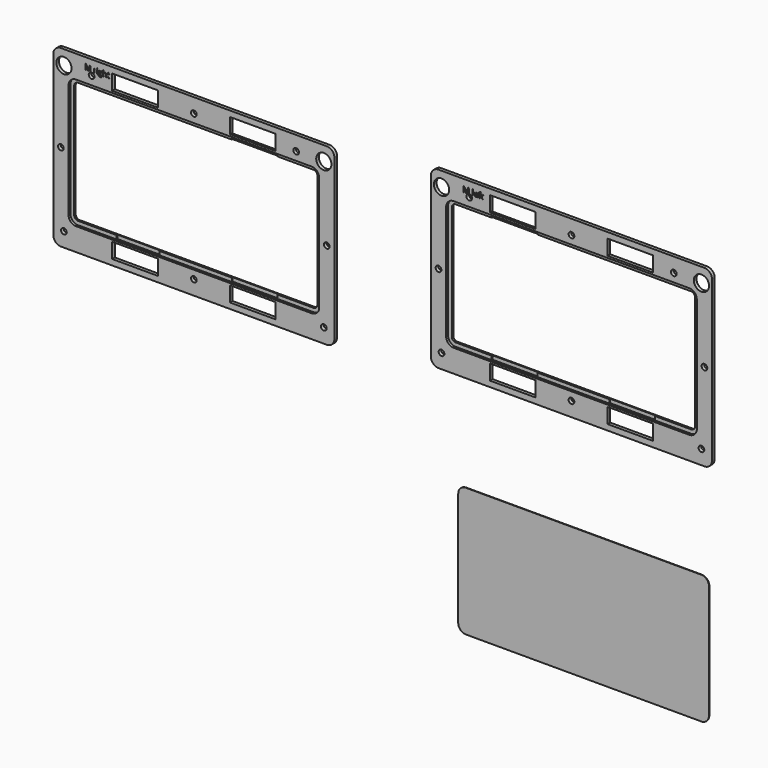
from build123d import *

# Parameters (mm, degrees)
F0_R          = 2.38125
F0_W          = 38.1
F0_H          = 12.7
F0_R_2        = 6.35
F0_R_3        = 2.3876
F1_DEPTH      = 0.79375
F2_R          = 2.38125
F2_W          = 38.1
F2_H          = 12.7
F2_R_2        = 6.35
F2_R_3        = 2.3876
F3_DEPTH      = 1.984375
F5_DEPTH      = 0.396875
F7_DEPTH      = 0.79375
F8_W          = 38.121374324
F8_H          = 5.2950307727
F9_DEPTH      = 0.79375
F10_TEXT_SIZE = 6.5434620612
F11_DEPTH     = 0.396875
F12_R         = 2.38125
F12_W         = 38.1
F12_H         = 12.7
F12_R_2       = 6.35
F12_R_3       = 2.3876
F13_DEPTH     = 0.79375
F14_R         = 2.38125
F14_W         = 38.1
F14_H         = 12.7
F14_R_2       = 6.35
F14_R_3       = 2.3876
F15_DEPTH     = 1.984375
F16_TEXT_SIZE = 6.2933967759
F17_DEPTH     = 0.396875
F19_DEPTH     = 0.79375
F20_W         = 38.1
F20_H         = 7.678820458
F20_H_2       = 9.2029287548
F20_W_2       = 35.9697821996
F20_H_3       = 10.6201223166
F21_DEPTH     = 0.79375


# Not quite as in the source:
# - Text() gives the source's letters only with a copy of the font that has no kerning and outlines rounded to 1/6400 em; it was checked with that copy


with BuildPart() as f1:
    # F0 (on Front) → F1 (new body)
    with BuildSketch(Plane.XZ):
        with BuildLine():
            Line((124.1159564874, 73.3042017429), (-98.1340435126, 73.3042017429))
            ThreePointArc((-98.1340435126, 73.3042017429), (-102.6241715732, 71.4443298034), (-104.4840435126, 66.9542017429))
            Line((-104.4840435126, 66.9542017429), (-104.4840435126, -66.3957982571))
            ThreePointArc((-104.4840435126, -66.3957982571), (-102.6241715732, -70.8859263176), (-98.1340435126, -72.7457982571))
            Line((-98.1340435126, -72.7457982571), (124.1159564874, -72.7457982571))
            ThreePointArc((124.1159564874, -72.7457982571), (128.6060845479, -70.8859263176), (130.4659564874, -66.3957982571))
            Line((130.4659564874, -66.3957982571), (130.4659564874, 66.9542017429))
            ThreePointArc((130.4659564874, 66.9542017429), (128.6060845479, 71.4443298034), (124.1159564874, 73.3042017429))
        make_face()
        with Locations((-95.6166075429, -60.7033622874)):
            Circle(F0_R, mode=Mode.SUBTRACT)
        with Locations((-36.2215435126, -61.6332982571)):
            Rectangle(F0_W, F0_H, mode=Mode.SUBTRACT)
        with Locations((12.994937633, -60.7033622874)):
            Circle(F0_R, mode=Mode.SUBTRACT)
        with Locations((62.2034564874, -61.6332982571)):
            Rectangle(F0_W, F0_H, mode=Mode.SUBTRACT)
        with Locations((121.5985205176, -60.7033622874)):
            Circle(F0_R, mode=Mode.SUBTRACT)
        with Locations((-98.1340435126, 0.2792017429)):
            Circle(F0_R, mode=Mode.SUBTRACT)
        with BuildLine():
            ThreePointArc((-91.7840435126, 47.9042017429), (-89.9241715732, 52.3943298034), (-85.4340435126, 54.2542017429))
            Line((-85.4340435126, 54.2542017429), (111.4159564874, 54.2542017429))
            ThreePointArc((111.4159564874, 54.2542017429), (115.9060845479, 52.3943298034), (117.7659564874, 47.9042017429))
            Line((117.7659564874, 47.9042017429), (117.7659564874, -47.3457982571))
            ThreePointArc((117.7659564874, -47.3457982571), (115.9060845479, -51.8359263176), (111.4159564874, -53.6957982571))
            Line((111.4159564874, -53.6957982571), (-85.4340435126, -53.6957982571))
            ThreePointArc((-85.4340435126, -53.6957982571), (-89.9241715732, -51.8359263176), (-91.7840435126, -47.3457982571))
            Line((-91.7840435126, -47.3457982571), (-91.7840435126, 47.9042017429))
        make_face(mode=Mode.SUBTRACT)
        with Locations((-95.6166075429, 61.2617657732)):
            Circle(F0_R_2, mode=Mode.SUBTRACT)
        with Locations((-72.4865459126, 61.2617657732)):
            Circle(F0_R_3, mode=Mode.SUBTRACT)
        with Locations((-36.2215435126, 62.1917017429)):
            Rectangle(F0_W, F0_H, mode=Mode.SUBTRACT)
        with Locations((124.1159564874, 0.2792017429)):
            Circle(F0_R, mode=Mode.SUBTRACT)
        with Locations((12.994937633, 61.2617657732)):
            Circle(F0_R, mode=Mode.SUBTRACT)
        with Locations((62.2034564874, 62.1917017429)):
            Rectangle(F0_W, F0_H, mode=Mode.SUBTRACT)
        with Locations((98.4684588874, 61.2617657732)):
            Circle(F0_R_3, mode=Mode.SUBTRACT)
        with Locations((121.5985205176, 61.2617657732)):
            Circle(F0_R_2, mode=Mode.SUBTRACT)
        with BuildLine():
            Line((111.4159564874, 54.2542017429), (-85.4340435126, 54.2542017429))
            ThreePointArc((-85.4340435126, 54.2542017429), (-89.9241715732, 52.3943298034), (-91.7840435126, 47.9042017429))
            Line((-91.7840435126, 47.9042017429), (-91.7840435126, -47.3457982571))
            ThreePointArc((-91.7840435126, -47.3457982571), (-89.9241715732, -51.8359263176), (-85.4340435126, -53.6957982571))
            Line((-85.4340435126, -53.6957982571), (111.4159564874, -53.6957982571))
            ThreePointArc((111.4159564874, -53.6957982571), (115.9060845479, -51.8359263176), (117.7659564874, -47.3457982571))
            Line((117.7659564874, -47.3457982571), (117.7659564874, 47.9042017429))
            ThreePointArc((117.7659564874, 47.9042017429), (115.9060845479, 52.3943298034), (111.4159564874, 54.2542017429))
        make_face()
        with BuildLine():
            ThreePointArc((-88.6090435126, 47.9042017429), (-87.6791075429, 50.1492657732), (-85.4340435126, 51.0792017429))
            Line((-85.4340435126, 51.0792017429), (111.4159564874, 51.0792017429))
            ThreePointArc((111.4159564874, 51.0792017429), (113.6610205176, 50.1492657732), (114.5909564874, 47.9042017429))
            Line((114.5909564874, 47.9042017429), (114.5909564874, -47.3457982571))
            ThreePointArc((114.5909564874, -47.3457982571), (113.6610205176, -49.5908622874), (111.4159564874, -50.5207982571))
            Line((111.4159564874, -50.5207982571), (-85.4340435126, -50.5207982571))
            ThreePointArc((-85.4340435126, -50.5207982571), (-87.6791075429, -49.5908622874), (-88.6090435126, -47.3457982571))
            Line((-88.6090435126, -47.3457982571), (-88.6090435126, 47.9042017429))
        make_face(mode=Mode.SUBTRACT)
    extrude(amount=F1_DEPTH)

    # F2 (on face) → F3 (join)
    with BuildSketch(Plane.XZ.offset(0.79375)):
        with BuildLine():
            ThreePointArc((124.1159564874, -72.7457982571), (128.6060845479, -70.8859263176), (130.4659564874, -66.3957982571))
            Line((130.4659564874, -66.3957982571), (130.4659564874, 66.9542017429))
            ThreePointArc((130.4659564874, 66.9542017429), (128.6060845479, 71.4443298034), (124.1159564874, 73.3042017429))
            Line((124.1159564874, 73.3042017429), (-98.1340435126, 73.3042017429))
            ThreePointArc((-98.1340435126, 73.3042017429), (-102.6241715732, 71.4443298034), (-104.4840435126, 66.9542017429))
            Line((-104.4840435126, 66.9542017429), (-104.4840435126, -66.3957982571))
            ThreePointArc((-104.4840435126, -66.3957982571), (-102.6241715732, -70.8859263176), (-98.1340435126, -72.7457982571))
            Line((-98.1340435126, -72.7457982571), (124.1159564874, -72.7457982571))
        make_face()
        with Locations((-95.6166075429, -60.7033622874)):
            Circle(F2_R, mode=Mode.SUBTRACT)
        with Locations((-36.2215435126, -61.6332982571)):
            Rectangle(F2_W, F2_H, mode=Mode.SUBTRACT)
        with Locations((12.994937633, -60.7033622874)):
            Circle(F2_R, mode=Mode.SUBTRACT)
        with Locations((62.2034564874, -61.6332982571)):
            Rectangle(F2_W, F2_H, mode=Mode.SUBTRACT)
        with Locations((121.5985205176, -60.7033622874)):
            Circle(F2_R, mode=Mode.SUBTRACT)
        with Locations((-98.1340435126, 0.2792017429)):
            Circle(F2_R, mode=Mode.SUBTRACT)
        with BuildLine():
            ThreePointArc((-91.7840435126, 47.9042017429), (-89.9241715732, 52.3943298034), (-85.4340435126, 54.2542017429))
            Line((-85.4340435126, 54.2542017429), (111.4159564874, 54.2542017429))
            ThreePointArc((111.4159564874, 54.2542017429), (115.9060845479, 52.3943298034), (117.7659564874, 47.9042017429))
            Line((117.7659564874, 47.9042017429), (117.7659564874, -47.3457982571))
            ThreePointArc((117.7659564874, -47.3457982571), (115.9060845479, -51.8359263176), (111.4159564874, -53.6957982571))
            Line((111.4159564874, -53.6957982571), (-85.4340435126, -53.6957982571))
            ThreePointArc((-85.4340435126, -53.6957982571), (-89.9241715732, -51.8359263176), (-91.7840435126, -47.3457982571))
            Line((-91.7840435126, -47.3457982571), (-91.7840435126, 47.9042017429))
        make_face(mode=Mode.SUBTRACT)
        with Locations((-95.6166075429, 61.2617657732)):
            Circle(F2_R_2, mode=Mode.SUBTRACT)
        with Locations((-72.4865459126, 61.2617657732)):
            Circle(F2_R_3, mode=Mode.SUBTRACT)
        with Locations((-36.2215435126, 62.1917017429)):
            Rectangle(F2_W, F2_H, mode=Mode.SUBTRACT)
        with Locations((124.1159564874, 0.2792017429)):
            Circle(F2_R, mode=Mode.SUBTRACT)
        with Locations((12.994937633, 61.2617657732)):
            Circle(F2_R, mode=Mode.SUBTRACT)
        with Locations((62.2034564874, 62.1917017429)):
            Rectangle(F2_W, F2_H, mode=Mode.SUBTRACT)
        with Locations((98.4684588874, 61.2617657732)):
            Circle(F2_R_3, mode=Mode.SUBTRACT)
        with Locations((121.5985205176, 61.2617657732)):
            Circle(F2_R_2, mode=Mode.SUBTRACT)
    extrude(amount=F3_DEPTH)

    # F6 (on face) → F7 (join)
    with BuildSketch(Plane(origin=(0, 0, 0), x_dir=(-1, 0, 0), z_dir=(0, 1, 0))):
        with BuildLine():
            ThreePointArc((91.7840435126, 47.9042017429), (89.9241715732, 52.3943298034), (85.4340435126, 54.2542017429))
            Line((85.4340435126, 54.2542017429), (55.2715435126, 54.2542017429))
            Line((55.2715435126, 54.2542017429), (17.1715435126, 54.2542017429))
            Line((17.1715435126, 54.2542017429), (-111.4159564874, 54.2542017429))
            ThreePointArc((-111.4159564874, 54.2542017429), (-115.9060845479, 52.3943298034), (-117.7659564874, 47.9042017429))
            Line((-117.7659564874, 47.9042017429), (-117.7659564874, -47.3457982571))
            ThreePointArc((-117.7659564874, -47.3457982571), (-115.9060845479, -51.8359263176), (-111.4159564874, -53.6957982571))
            Line((-111.4159564874, -53.6957982571), (85.4340435126, -53.6957982571))
            ThreePointArc((85.4340435126, -53.6957982571), (89.9241715732, -51.8359263176), (91.7840435126, -47.3457982571))
            Line((91.7840435126, -47.3457982571), (91.7840435126, 47.9042017429))
        make_face()
        with BuildLine():
            Line((-111.4159564874, 51.0792017429), (85.4340435126, 51.0792017429))
            ThreePointArc((85.4340435126, 51.0792017429), (87.6791075429, 50.1492657732), (88.6090435126, 47.9042017429))
            Line((88.6090435126, 47.9042017429), (88.6090435126, -47.3457982571))
            ThreePointArc((88.6090435126, -47.3457982571), (87.6791075429, -49.5908622874), (85.4340435126, -50.5207982571))
            Line((85.4340435126, -50.5207982571), (-111.4159564874, -50.5207982571))
            ThreePointArc((-111.4159564874, -50.5207982571), (-113.6610205176, -49.5908622874), (-114.5909564874, -47.3457982571))
            Line((-114.5909564874, -47.3457982571), (-114.5909564874, 47.9042017429))
            ThreePointArc((-114.5909564874, 47.9042017429), (-113.6610205176, 50.1492657732), (-111.4159564874, 51.0792017429))
        make_face(mode=Mode.SUBTRACT)
    extrude(amount=F7_DEPTH)

    # F8 (on face) → F9 (cut)
    with BuildSketch(Plane.XZ):
        with Locations((-36.2322209403, 53.1942471862)):
            Rectangle(F8_W, F8_H)
        with Locations((-36.2322209403, -52.6358437004)):
            Rectangle(F8_W, F8_H)
        with Locations((62.214133915, -52.6358437004)):
            Rectangle(F8_W, F8_H)
    extrude(amount=F9_DEPTH, mode=Mode.SUBTRACT)

    # F10 (on face) → F11 (cut)
    with BuildSketch(Plane.XZ.offset(2.778125)):
        with Locations((-77.8341839889, 63.4480455194)):
            Text('M left', F10_TEXT_SIZE, font='Open Sans', text_align=(TextAlign.LEFT, TextAlign.BOTTOM))
    extrude(amount=-F11_DEPTH, mode=Mode.SUBTRACT)


with BuildPart() as f5:
    # F4 (on Front) → F5 (new body)
    with BuildSketch(Plane.XZ):
        with BuildLine():
            Line((119.6384238243, -154.9380476216), (-77.2115761757, -154.9380476216))
            ThreePointArc((-77.2115761757, -154.9380476216), (-81.7017042362, -156.7979195611), (-83.5615761757, -161.2880476216))
            Line((-83.5615761757, -161.2880476216), (-83.5615761757, -256.5380476216))
            ThreePointArc((-83.5615761757, -256.5380476216), (-81.7017042362, -261.0281756821), (-77.2115761757, -262.8880476216))
            Line((-77.2115761757, -262.8880476216), (119.6384238243, -262.8880476216))
            ThreePointArc((119.6384238243, -262.8880476216), (124.1285518848, -261.0281756821), (125.9884238243, -256.5380476216))
            Line((125.9884238243, -256.5380476216), (125.9884238243, -161.2880476216))
            ThreePointArc((125.9884238243, -161.2880476216), (124.1285518848, -156.7979195611), (119.6384238243, -154.9380476216))
        make_face()
    extrude(amount=F5_DEPTH)


with BuildPart() as f13:
    # F12 (on Front) → F13 (new body)
    with BuildSketch(Plane.XZ):
        with BuildLine():
            Line((-191.4938860515, 60.1202354639), (-413.7438860515, 60.1202354639))
            ThreePointArc((-413.7438860515, 60.1202354639), (-418.234014112, 58.2603635244), (-420.0938860515, 53.7702354639))
            Line((-420.0938860515, 53.7702354639), (-420.0938860515, -79.5797645361))
            ThreePointArc((-420.0938860515, -79.5797645361), (-418.234014112, -84.0698925967), (-413.7438860515, -85.9297645361))
            Line((-413.7438860515, -85.9297645361), (-191.4938860515, -85.9297645361))
            ThreePointArc((-191.4938860515, -85.9297645361), (-187.0037579909, -84.0698925967), (-185.1438860515, -79.5797645361))
            Line((-185.1438860515, -79.5797645361), (-185.1438860515, 53.7702354639))
            ThreePointArc((-185.1438860515, 53.7702354639), (-187.0037579909, 58.2603635244), (-191.4938860515, 60.1202354639))
        make_face()
        with Locations((-411.2264500817, -73.8873285664)):
            Circle(F12_R, mode=Mode.SUBTRACT)
        with Locations((-351.8313860515, -74.8172645361)):
            Rectangle(F12_W, F12_H, mode=Mode.SUBTRACT)
        with Locations((-413.7438860515, -12.9047645361)):
            Circle(F12_R, mode=Mode.SUBTRACT)
        with BuildLine():
            ThreePointArc((-407.3938860515, 34.7202354639), (-405.534014112, 39.2103635244), (-401.0438860515, 41.0702354639))
            Line((-401.0438860515, 41.0702354639), (-204.1938860515, 41.0702354639))
            ThreePointArc((-204.1938860515, 41.0702354639), (-199.7037579909, 39.2103635244), (-197.8438860515, 34.7202354639))
            Line((-197.8438860515, 34.7202354639), (-197.8438860515, -60.5297645361))
            ThreePointArc((-197.8438860515, -60.5297645361), (-199.7037579909, -65.0198925967), (-204.1938860515, -66.8797645361))
            Line((-204.1938860515, -66.8797645361), (-401.0438860515, -66.8797645361))
            ThreePointArc((-401.0438860515, -66.8797645361), (-405.534014112, -65.0198925967), (-407.3938860515, -60.5297645361))
            Line((-407.3938860515, -60.5297645361), (-407.3938860515, 34.7202354639))
        make_face(mode=Mode.SUBTRACT)
        with Locations((-302.6149049058, -73.8873285664)):
            Circle(F12_R, mode=Mode.SUBTRACT)
        with Locations((-253.4063860515, -74.8172645361)):
            Rectangle(F12_W, F12_H, mode=Mode.SUBTRACT)
        with Locations((-194.0113220212, -73.8873285664)):
            Circle(F12_R, mode=Mode.SUBTRACT)
        with Locations((-191.4938860515, -12.9047645361)):
            Circle(F12_R, mode=Mode.SUBTRACT)
        with Locations((-411.2264500817, 48.0777994941)):
            Circle(F12_R_2, mode=Mode.SUBTRACT)
        with Locations((-388.0963884515, 48.0777994941)):
            Circle(F12_R_3, mode=Mode.SUBTRACT)
        with Locations((-351.8313860515, 49.0077354639)):
            Rectangle(F12_W, F12_H, mode=Mode.SUBTRACT)
        with Locations((-302.6149049058, 48.0777994941)):
            Circle(F12_R, mode=Mode.SUBTRACT)
        with Locations((-253.4063860515, 49.0077354639)):
            Rectangle(F12_W, F12_H, mode=Mode.SUBTRACT)
        with Locations((-217.1413836515, 48.0777994941)):
            Circle(F12_R_3, mode=Mode.SUBTRACT)
        with Locations((-194.0113220212, 48.0777994941)):
            Circle(F12_R_2, mode=Mode.SUBTRACT)
        with BuildLine():
            Line((-204.1938860515, 41.0702354639), (-401.0438860515, 41.0702354639))
            ThreePointArc((-401.0438860515, 41.0702354639), (-405.534014112, 39.2103635244), (-407.3938860515, 34.7202354639))
            Line((-407.3938860515, 34.7202354639), (-407.3938860515, -60.5297645361))
            ThreePointArc((-407.3938860515, -60.5297645361), (-405.534014112, -65.0198925967), (-401.0438860515, -66.8797645361))
            Line((-401.0438860515, -66.8797645361), (-204.1938860515, -66.8797645361))
            ThreePointArc((-204.1938860515, -66.8797645361), (-199.7037579909, -65.0198925967), (-197.8438860515, -60.5297645361))
            Line((-197.8438860515, -60.5297645361), (-197.8438860515, 34.7202354639))
            ThreePointArc((-197.8438860515, 34.7202354639), (-199.7037579909, 39.2103635244), (-204.1938860515, 41.0702354639))
        make_face()
        with BuildLine():
            ThreePointArc((-404.2188860515, 34.7202354639), (-403.2889500817, 36.9652994941), (-401.0438860515, 37.8952354639))
            Line((-401.0438860515, 37.8952354639), (-204.1938860515, 37.8952354639))
            ThreePointArc((-204.1938860515, 37.8952354639), (-201.9488220212, 36.9652994941), (-201.0188860515, 34.7202354639))
            Line((-201.0188860515, 34.7202354639), (-201.0188860515, -60.5297645361))
            ThreePointArc((-201.0188860515, -60.5297645361), (-201.9488220212, -62.7748285664), (-204.1938860515, -63.7047645361))
            Line((-204.1938860515, -63.7047645361), (-401.0438860515, -63.7047645361))
            ThreePointArc((-401.0438860515, -63.7047645361), (-403.2889500817, -62.7748285664), (-404.2188860515, -60.5297645361))
            Line((-404.2188860515, -60.5297645361), (-404.2188860515, 34.7202354639))
        make_face(mode=Mode.SUBTRACT)
    extrude(amount=F13_DEPTH)

    # F14 (on face) → F15 (join)
    with BuildSketch(Plane.XZ.offset(0.79375)):
        with BuildLine():
            ThreePointArc((-185.1438860515, 53.7702354639), (-187.0037579909, 58.2603635244), (-191.4938860515, 60.1202354639))
            Line((-191.4938860515, 60.1202354639), (-413.7438860515, 60.1202354639))
            ThreePointArc((-413.7438860515, 60.1202354639), (-418.234014112, 58.2603635244), (-420.0938860515, 53.7702354639))
            Line((-420.0938860515, 53.7702354639), (-420.0938860515, -79.5797645361))
            ThreePointArc((-420.0938860515, -79.5797645361), (-418.234014112, -84.0698925967), (-413.7438860515, -85.9297645361))
            Line((-413.7438860515, -85.9297645361), (-191.4938860515, -85.9297645361))
            ThreePointArc((-191.4938860515, -85.9297645361), (-187.0037579909, -84.0698925967), (-185.1438860515, -79.5797645361))
            Line((-185.1438860515, -79.5797645361), (-185.1438860515, 53.7702354639))
        make_face()
        with Locations((-411.2264500817, -73.8873285664)):
            Circle(F14_R, mode=Mode.SUBTRACT)
        with Locations((-351.8313860515, -74.8172645361)):
            Rectangle(F14_W, F14_H, mode=Mode.SUBTRACT)
        with BuildLine():
            ThreePointArc((-407.3938860515, 34.7202354639), (-405.534014112, 39.2103635244), (-401.0438860515, 41.0702354639))
            Line((-401.0438860515, 41.0702354639), (-204.1938860515, 41.0702354639))
            ThreePointArc((-204.1938860515, 41.0702354639), (-199.7037579909, 39.2103635244), (-197.8438860515, 34.7202354639))
            Line((-197.8438860515, 34.7202354639), (-197.8438860515, -60.5297645361))
            ThreePointArc((-197.8438860515, -60.5297645361), (-199.7037579909, -65.0198925967), (-204.1938860515, -66.8797645361))
            Line((-204.1938860515, -66.8797645361), (-401.0438860515, -66.8797645361))
            ThreePointArc((-401.0438860515, -66.8797645361), (-405.534014112, -65.0198925967), (-407.3938860515, -60.5297645361))
            Line((-407.3938860515, -60.5297645361), (-407.3938860515, 34.7202354639))
        make_face(mode=Mode.SUBTRACT)
        with Locations((-302.6149049058, -73.8873285664)):
            Circle(F14_R, mode=Mode.SUBTRACT)
        with Locations((-253.4063860515, -74.8172645361)):
            Rectangle(F14_W, F14_H, mode=Mode.SUBTRACT)
        with Locations((-194.0113220212, -73.8873285664)):
            Circle(F14_R, mode=Mode.SUBTRACT)
        with Locations((-413.7438860515, -12.9047645361)):
            Circle(F14_R, mode=Mode.SUBTRACT)
        with Locations((-411.2264500817, 48.0777994941)):
            Circle(F14_R_2, mode=Mode.SUBTRACT)
        with Locations((-388.0963884515, 48.0777994941)):
            Circle(F14_R_3, mode=Mode.SUBTRACT)
        with Locations((-351.8313860515, 49.0077354639)):
            Rectangle(F14_W, F14_H, mode=Mode.SUBTRACT)
        with Locations((-191.4938860515, -12.9047645361)):
            Circle(F14_R, mode=Mode.SUBTRACT)
        with Locations((-302.6149049058, 48.0777994941)):
            Circle(F14_R, mode=Mode.SUBTRACT)
        with Locations((-253.4063860515, 49.0077354639)):
            Rectangle(F14_W, F14_H, mode=Mode.SUBTRACT)
        with Locations((-217.1413836515, 48.0777994941)):
            Circle(F14_R_3, mode=Mode.SUBTRACT)
        with Locations((-194.0113220212, 48.0777994941)):
            Circle(F14_R_2, mode=Mode.SUBTRACT)
    extrude(amount=F15_DEPTH)

    # F16 (on face) → F17 (cut)
    with BuildSketch(Plane.XZ.offset(2.778125)):
        with Locations((-393.8792347908, 50.8477687836)):
            Text('M right', F16_TEXT_SIZE, font='Open Sans', text_align=(TextAlign.LEFT, TextAlign.BOTTOM))
    extrude(amount=-F17_DEPTH, mode=Mode.SUBTRACT)

    # F18 (on face) → F19 (join)
    with BuildSketch(Plane(origin=(0, 0, 0), x_dir=(-1, 0, 0), z_dir=(0, 1, 0))):
        with BuildLine():
            ThreePointArc((407.3938860515, 34.7202354639), (405.534014112, 39.2103635244), (401.0438860515, 41.0702354639))
            Line((401.0438860515, 41.0702354639), (204.1938860515, 41.0702354639))
            ThreePointArc((204.1938860515, 41.0702354639), (199.7037579909, 39.2103635244), (197.8438860515, 34.7202354639))
            Line((197.8438860515, 34.7202354639), (197.8438860515, -60.5297645361))
            ThreePointArc((197.8438860515, -60.5297645361), (199.7037579909, -65.0198925967), (204.1938860515, -66.8797645361))
            Line((204.1938860515, -66.8797645361), (401.0438860515, -66.8797645361))
            ThreePointArc((401.0438860515, -66.8797645361), (405.534014112, -65.0198925967), (407.3938860515, -60.5297645361))
            Line((407.3938860515, -60.5297645361), (407.3938860515, 34.7202354639))
        make_face()
        with BuildLine():
            Line((204.1938860515, 37.8952354639), (401.0438860515, 37.8952354639))
            ThreePointArc((401.0438860515, 37.8952354639), (403.2889500817, 36.9652994941), (404.2188860515, 34.7202354639))
            Line((404.2188860515, 34.7202354639), (404.2188860515, -60.5297645361))
            ThreePointArc((404.2188860515, -60.5297645361), (403.2889500817, -62.7748285664), (401.0438860515, -63.7047645361))
            Line((401.0438860515, -63.7047645361), (204.1938860515, -63.7047645361))
            ThreePointArc((204.1938860515, -63.7047645361), (201.9488220212, -62.7748285664), (201.0188860515, -60.5297645361))
            Line((201.0188860515, -60.5297645361), (201.0188860515, 34.7202354639))
            ThreePointArc((201.0188860515, 34.7202354639), (201.9488220212, 36.9652994941), (204.1938860515, 37.8952354639))
        make_face(mode=Mode.SUBTRACT)
    extrude(amount=F19_DEPTH)

    # F20 (on face) → F21 (cut)
    with BuildSketch(Plane(origin=(0, 0, 0), x_dir=(-1, 0, 0), z_dir=(0, 1, 0))):
        with Locations((253.4063860515, 38.8183252349)):
            Rectangle(F20_W, F20_H)
        with Locations((253.4063860515, -63.8658001587)):
            Rectangle(F20_W, F20_H_2)
        with Locations((350.7662771513, -63.1572033778)):
            Rectangle(F20_W_2, F20_H_3)
    extrude(amount=-F21_DEPTH, mode=Mode.SUBTRACT)


solid = Compound([f1.part, f5.part, f13.part])
